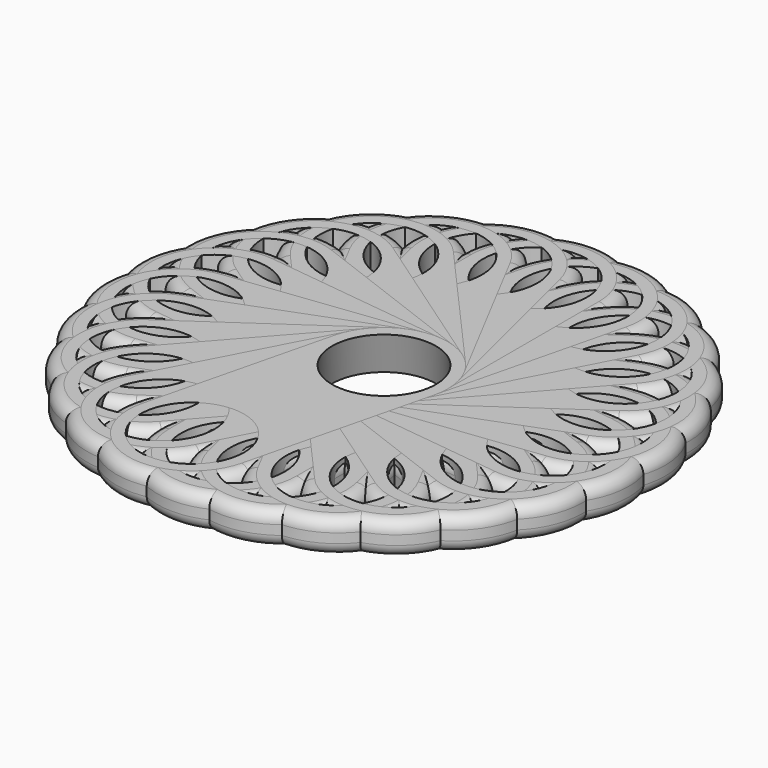
from build123d import *

# Parameters (mm, degrees)
F1_DEPTH = 7
F2_R     = 11
F3_DEPTH = 7.001
F5_R     = 2.5
F6_R     = 2.5
F7_COUNT = 26


with BuildPart() as f1:
    # F0 (on Top) → F1 (new body)
    with BuildSketch(Plane.XY):
        with BuildLine():
            ThreePointArc((-16, 0), (0, -16), (16, 0))
            ThreePointArc((16, 0), (0, 16), (-16, 0))
        make_face()
        with BuildLine():
            Line((16, -40), (16, 0))
            ThreePointArc((16, 0), (0, -16), (-16, 0))
            Line((-16, 0), (-16, -40))
            ThreePointArc((-16, -40), (0, -24), (16, -40))
        make_face()
        with BuildLine():
            ThreePointArc((-16, -40), (0, -56), (16, -40))
            ThreePointArc((16, -40), (0, -24), (-16, -40))
        make_face()
    extrude(amount=-F1_DEPTH)

    # F2 (on Top) → F3 (cut, through all)
    with BuildSketch(Plane.XY):
        Circle(F2_R)
        with Locations((0, -40)):
            Circle(F2_R)
    extrude(amount=-F3_DEPTH, mode=Mode.SUBTRACT)

    # F5
    f5_edges = [f1.edges().sort_by_distance(p)[0] for p in [
        (0, -56, 0),
    ]]
    fillet(f5_edges, radius=F5_R)

    # F6
    f6_edges = [f1.edges().sort_by_distance(p)[0] for p in [
        (0, -56, -7),
    ]]
    fillet(f6_edges, radius=F6_R)


with BuildPart() as f7_1:
    # F7: instance of F1
    add(f1.part.rotate(Axis((0, 0, 24.5344247669), (0, 0, 1)), 1 * 360 / F7_COUNT))


with BuildPart() as f7_2:
    # F7: instance of F1
    add(f1.part.rotate(Axis((0, 0, 24.5344247669), (0, 0, 1)), 2 * 360 / F7_COUNT))


with BuildPart() as f7_3:
    # F7: instance of F1
    add(f1.part.rotate(Axis((0, 0, 24.5344247669), (0, 0, 1)), 3 * 360 / F7_COUNT))


with BuildPart() as f7_4:
    # F7: instance of F1
    add(f1.part.rotate(Axis((0, 0, 24.5344247669), (0, 0, 1)), 4 * 360 / F7_COUNT))


with BuildPart() as f7_5:
    # F7: instance of F1
    add(f1.part.rotate(Axis((0, 0, 24.5344247669), (0, 0, 1)), 5 * 360 / F7_COUNT))


with BuildPart() as f7_6:
    # F7: instance of F1
    add(f1.part.rotate(Axis((0, 0, 24.5344247669), (0, 0, 1)), 6 * 360 / F7_COUNT))


with BuildPart() as f7_7:
    # F7: instance of F1
    add(f1.part.rotate(Axis((0, 0, 24.5344247669), (0, 0, 1)), 7 * 360 / F7_COUNT))


with BuildPart() as f7_8:
    # F7: instance of F1
    add(f1.part.rotate(Axis((0, 0, 24.5344247669), (0, 0, 1)), 8 * 360 / F7_COUNT))


with BuildPart() as f7_9:
    # F7: instance of F1
    add(f1.part.rotate(Axis((0, 0, 24.5344247669), (0, 0, 1)), 9 * 360 / F7_COUNT))


with BuildPart() as f7_10:
    # F7: instance of F1
    add(f1.part.rotate(Axis((0, 0, 24.5344247669), (0, 0, 1)), 10 * 360 / F7_COUNT))


with BuildPart() as f7_11:
    # F7: instance of F1
    add(f1.part.rotate(Axis((0, 0, 24.5344247669), (0, 0, 1)), 11 * 360 / F7_COUNT))


with BuildPart() as f7_12:
    # F7: instance of F1
    add(f1.part.rotate(Axis((0, 0, 24.5344247669), (0, 0, 1)), 12 * 360 / F7_COUNT))


with BuildPart() as f7_13:
    # F7: instance of F1
    add(f1.part.rotate(Axis((0, 0, 24.5344247669), (0, 0, 1)), 13 * 360 / F7_COUNT))


with BuildPart() as f7_14:
    # F7: instance of F1
    add(f1.part.rotate(Axis((0, 0, 24.5344247669), (0, 0, 1)), 14 * 360 / F7_COUNT))


with BuildPart() as f7_15:
    # F7: instance of F1
    add(f1.part.rotate(Axis((0, 0, 24.5344247669), (0, 0, 1)), 15 * 360 / F7_COUNT))


with BuildPart() as f7_16:
    # F7: instance of F1
    add(f1.part.rotate(Axis((0, 0, 24.5344247669), (0, 0, 1)), 16 * 360 / F7_COUNT))


with BuildPart() as f7_17:
    # F7: instance of F1
    add(f1.part.rotate(Axis((0, 0, 24.5344247669), (0, 0, 1)), 17 * 360 / F7_COUNT))


with BuildPart() as f7_18:
    # F7: instance of F1
    add(f1.part.rotate(Axis((0, 0, 24.5344247669), (0, 0, 1)), 18 * 360 / F7_COUNT))


with BuildPart() as f7_19:
    # F7: instance of F1
    add(f1.part.rotate(Axis((0, 0, 24.5344247669), (0, 0, 1)), 19 * 360 / F7_COUNT))


with BuildPart() as f7_20:
    # F7: instance of F1
    add(f1.part.rotate(Axis((0, 0, 24.5344247669), (0, 0, 1)), 20 * 360 / F7_COUNT))


with BuildPart() as f7_21:
    # F7: instance of F1
    add(f1.part.rotate(Axis((0, 0, 24.5344247669), (0, 0, 1)), 21 * 360 / F7_COUNT))


with BuildPart() as f7_22:
    # F7: instance of F1
    add(f1.part.rotate(Axis((0, 0, 24.5344247669), (0, 0, 1)), 22 * 360 / F7_COUNT))


with BuildPart() as f7_23:
    # F7: instance of F1
    add(f1.part.rotate(Axis((0, 0, 24.5344247669), (0, 0, 1)), 23 * 360 / F7_COUNT))


with BuildPart() as f7_24:
    # F7: instance of F1
    add(f1.part.rotate(Axis((0, 0, 24.5344247669), (0, 0, 1)), 24 * 360 / F7_COUNT))


with BuildPart() as f7_25:
    # F7: instance of F1
    add(f1.part.rotate(Axis((0, 0, 24.5344247669), (0, 0, 1)), 25 * 360 / F7_COUNT))


solid = Compound([f1.part, f7_1.part, f7_2.part, f7_3.part, f7_4.part, f7_5.part, f7_6.part, f7_7.part, f7_8.part, f7_9.part, f7_10.part, f7_11.part, f7_12.part, f7_13.part, f7_14.part, f7_15.part, f7_16.part, f7_17.part, f7_18.part, f7_19.part, f7_20.part, f7_21.part, f7_22.part, f7_23.part, f7_24.part, f7_25.part])
